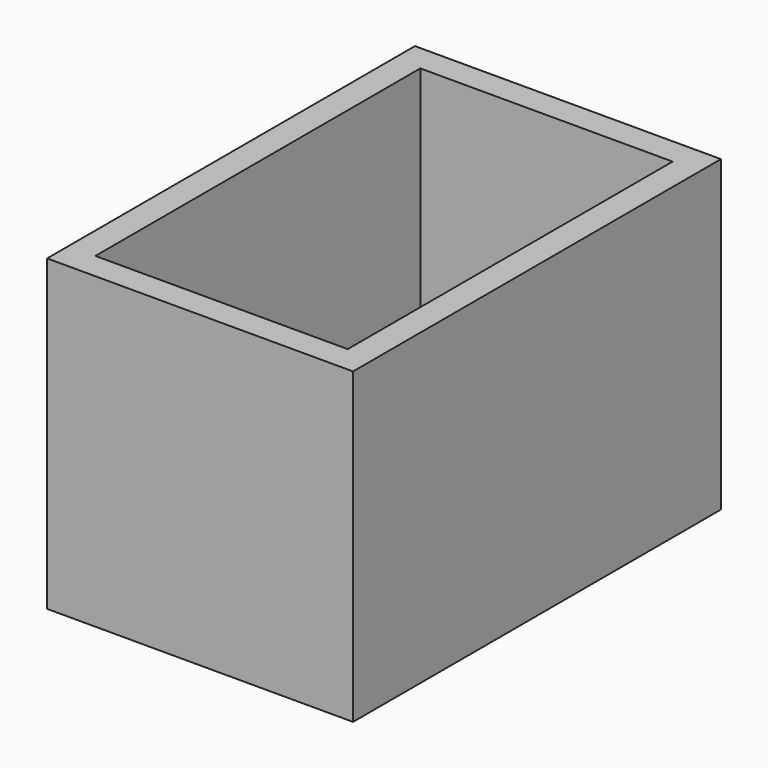
from build123d import *

# Parameters (mm, degrees)
F1_W     = 28.9652645588
F1_H     = 43.5288026929
F2_DEPTH = 3.81
F3_DEPTH = 25.4
F4_T     = -2.54


# Not quite as in the source:
# - a feature of the source that left no trace in its solid (it failed there, or was rolled back) is left out


with BuildPart() as f2:
    # F1 (on Top) → F2 (new body)
    with BuildSketch(Plane.XY):
        with Locations((29.5196138322, -1.5338174999)):
            Rectangle(F1_W, F1_H)
    extrude(amount=F2_DEPTH)

    # F3 (add): a face of the model
    f3_faces = [f2.faces().sort_by_distance(p)[0] for p in [
        (29.5196138322, -1.5338174999, 3.81),
    ]]
    extrude(f3_faces, amount=F3_DEPTH)

    # F4
    f4_openings = [f2.faces().sort_by_distance(p)[0] for p in [
        (29.519614, -1.533817, 29.21),
    ]]
    offset(amount=F4_T, openings=f4_openings)


solid = f2.part
